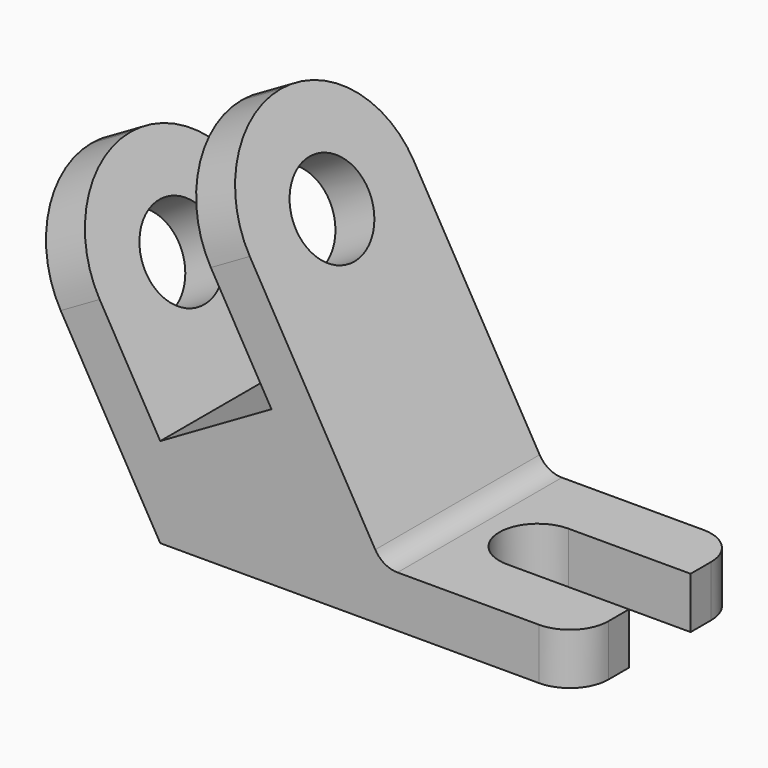
from build123d import *

# Parameters (mm, degrees)
F1_DEPTH = 25.4
F3_DEPTH = 12.701
F5_D     = 22.225
F6_R     = 25.39999
F7_R     = 9.525


# Not quite as in the source:
# - a fillet or chamfer is up to 0.001 mm smaller than in the source, because OpenCascade refuses the exact size


with BuildPart() as f1:
    # F0 (on Front) → F1 (new body, symmetric)
    with BuildSketch(Plane.XZ):
        with BuildLine():
            Line((-37.30625, 64.6163204399), (0, 0))
            Line((0, 0), (103.1875, 0))
            Line((103.1875, 0), (103.1875, 12.7))
            Line((103.1875, 12.7), (58.6587873497, 12.7))
            ThreePointArc((58.6587873497, 12.7), (55.4837873497, 13.550738686), (53.1595260356, 15.875))
            Line((53.1595260356, 15.875), (9.4374711693, 91.6038204399))
            Line((9.4374711693, 91.6038204399), (-0.1862361303, 86.0475704399))
            Line((-0.1862361303, 86.0475704399), (27.4963065702, 38.1))
            Line((27.4963065702, 38.1), (0, 22.225))
            Line((0, 22.225), (-27.6825427004, 70.1725704399))
            Line((-27.6825427004, 70.1725704399), (-37.30625, 64.6163204399))
        make_face()
    extrude(amount=F1_DEPTH, both=True)

    # F2 (on face) → F3 (cut, through all)
    with BuildSketch(Plane.XY.offset(12.7)):
        with BuildLine():
            Line((103.1875, 9.525), (73.025, 9.525))
            ThreePointArc((73.025, 9.525), (63.5, 0), (73.025, -9.525))
            Line((73.025, -9.525), (103.1875, -9.525))
            Line((103.1875, -9.525), (103.1875, 9.525))
        make_face()
    extrude(amount=-F3_DEPTH, mode=Mode.SUBTRACT)

    # F5 (through all)
    with Locations(Plane(origin=(46.7437211693, 0, 26.9875), x_dir=(0, 1, 0), z_dir=(0.8660254038, 0, 0.5))):
        with Locations((0, 49.2125)):
            Hole(F5_D / 2)

    # F6 (radius 25.4 in the source; OpenCascade refuses exactly that, so slightly less here)
    f6_edges = [f1.edges().sort_by_distance(p)[0] for p in [
        (-32.494396, 25.4, 67.394445),
        (4.625618, 25.4, 88.825695),
        (-32.494396, -25.4, 67.394445),
        (4.625618, -25.4, 88.825695),
    ]]
    fillet(f6_edges, radius=F6_R)

    # F7
    f7_edges = [f1.edges().sort_by_distance(p)[0] for p in [
        (103.1875, 25.4, 6.35),
        (103.1875, -25.4, 6.35),
    ]]
    fillet(f7_edges, radius=F7_R)


solid = f1.part
